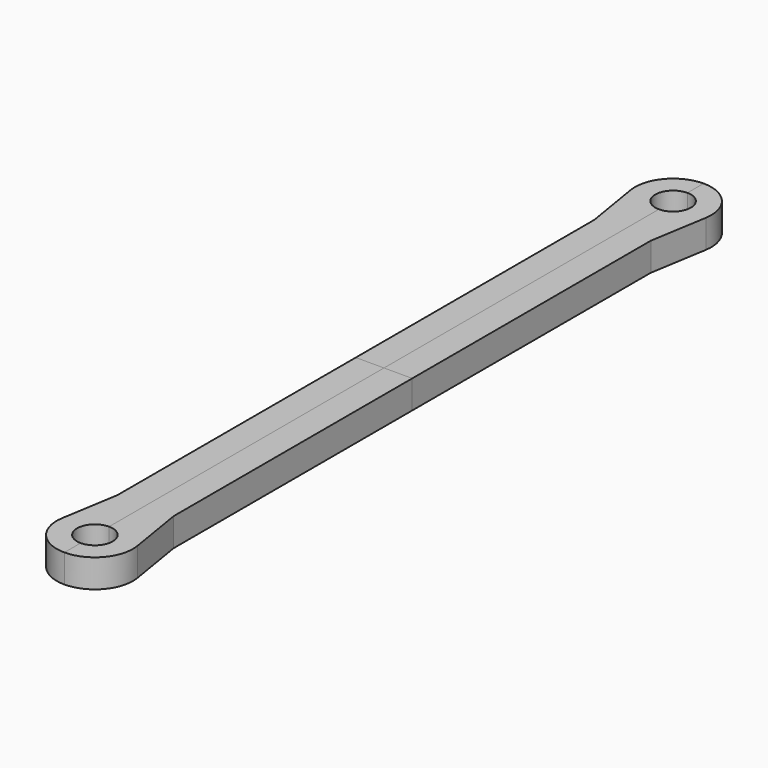
from build123d import *
from build123d import SkipClean  # not in build123d's __all__

# Parameters (mm, degrees)
F1_DEPTH = 3.175


with BuildPart() as f1:
    # F0 (on Top) → F1 (new body, symmetric)
    with BuildSketch(Plane.XY):
        with BuildLine():
            ThreePointArc((0, -77.28), (4, -81.28), (0, -85.28))
            Line((0, -85.28), (0, -89.8525))
            ThreePointArc((0, -89.8525), (6.5348908987, -86.8282391073), (8.4589413231, -79.8892922874))
            Line((8.4589413231, -79.8892922874), (6.35, -67.061714828))
            Line((6.35, -67.061714828), (6.35, 0))
            Line((6.35, 0), (0, 0))
            Line((0, 0), (0, -77.28))
        make_face()
    extrude(amount=F1_DEPTH, both=True)

    # F2: F1 across plane


with BuildPart() as f1_1:
    add(f1.part, clean=False)
    with SkipClean():  # cleaning this boolean's faces spoils the solid; the shape is the same uncleaned
        add(f1.part.mirror(Plane.YZ), clean=False)

    # F3: F1 across plane


with BuildPart() as f1_2:
    add(f1_1.part, clean=False)
    add(f1_1.part.mirror(Plane.XZ), clean=False)


solid = f1_2.part
